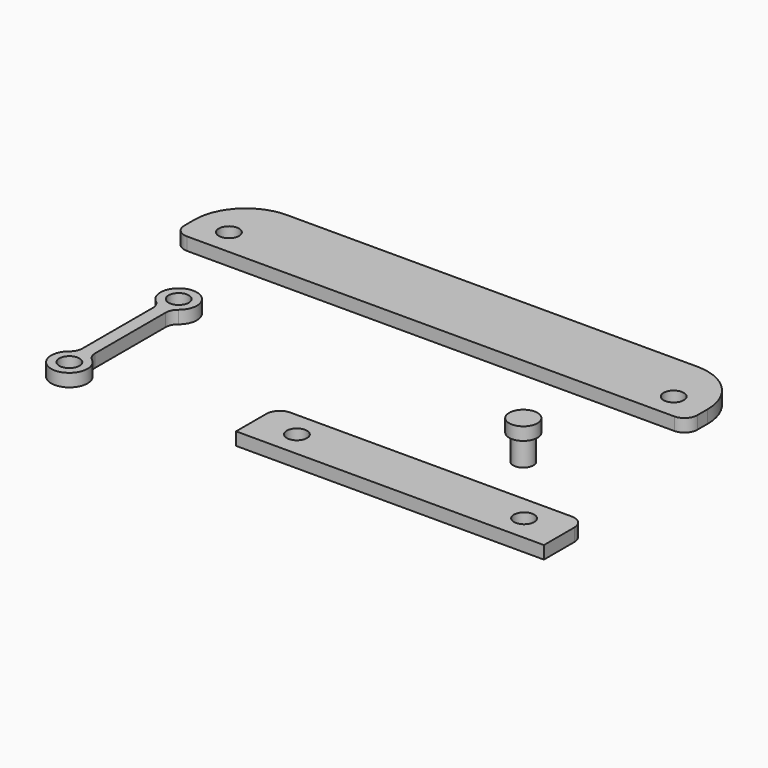
from build123d import *

# Parameters (mm, degrees)
F0_R     = 2.5
F1_DEPTH = 3.175
F2_R     = 2.5
F3_DEPTH = 3.175
F4_R     = 2.5
F5_DEPTH = 6.35
F4_R_2   = 3.5
F6_DEPTH = 3.175
F8_DEPTH = 3.175


# Not quite as in the source:
# - a length typed as a fraction of an inch, garbled in the dataset ("3 / 203.2 mm" for 3/8 in), is restored


with BuildPart() as f1:
    # F0 (on Top) → F1 (new body)
    with BuildSketch(Plane.XY):
        with BuildLine():
            ThreePointArc((-33.712554723, 10.891355979), (-33.3953284467, 12.2747410823), (-32.5070401756, 13.3816876943))
            ThreePointArc((-32.5070401756, 13.3816876943), (-35.2984368801, 21.4112917002), (-38.0898335846, 13.3816876943))
            ThreePointArc((-38.0898335846, 13.3816876943), (-37.2015453135, 12.2747410823), (-36.8843190372, 10.891355979))
            Line((-36.8843190372, 10.891355979), (-36.8843190372, 0))
            Line((-36.8843190372, 0), (-33.712554723, 0))
            Line((-33.712554723, 0), (-33.712554723, 10.891355979))
        make_face()
        with Locations((-35.2984368801, 16.9112917002)):
            Circle(F0_R, mode=Mode.SUBTRACT)
        with BuildLine():
            Line((-33.712554723, -10.891355979), (-33.712554723, 0))
            Line((-33.712554723, 0), (-36.8843190372, 0))
            Line((-36.8843190372, 0), (-36.8843190372, -10.891355979))
            ThreePointArc((-36.8843190372, -10.891355979), (-37.2015453135, -12.2747410823), (-38.0898335846, -13.3816876943))
            ThreePointArc((-38.0898335846, -13.3816876943), (-35.2984368801, -21.4112917002), (-32.5070401756, -13.3816876943))
            ThreePointArc((-32.5070401756, -13.3816876943), (-33.3953284467, -12.2747410823), (-33.712554723, -10.891355979))
        make_face()
        with Locations((-35.2984368801, -16.9112917002)):
            Circle(F0_R, mode=Mode.SUBTRACT)
    extrude(amount=F1_DEPTH)


with BuildPart() as f3:
    # F2 (on Top) → F3 (new body)
    with BuildSketch(Plane.XY):
        with BuildLine():
            ThreePointArc((-53.6429062486, 41.5569074162), (-52.7129702788, 39.3118433859), (-50.4679062486, 38.3819074162))
            Line((-50.4679062486, 38.3819074162), (9.8570937514, 38.3819074162))
            Line((9.8570937514, 38.3819074162), (70.1820937514, 38.3819074162))
            ThreePointArc((70.1820937514, 38.3819074162), (72.4271577817, 39.3118433859), (73.3570937514, 41.5569074162))
            Line((73.3570937514, 41.5569074162), (73.3570937514, 44.7319074162))
            ThreePointArc((73.3570937514, 44.7319074162), (69.6373498725, 53.7121635373), (60.6570937514, 57.4319074162))
            Line((60.6570937514, 57.4319074162), (9.8570937514, 57.4319074162))
            Line((9.8570937514, 57.4319074162), (-40.9429062486, 57.4319074162))
            ThreePointArc((-40.9429062486, 57.4319074162), (-49.9231623696, 53.7121635373), (-53.6429062486, 44.7319074162))
            Line((-53.6429062486, 44.7319074162), (-53.6429062486, 41.5569074162))
        make_face()
        with Locations((-45.1785493704, 44.8088147985)):
            Circle(F2_R, mode=Mode.SUBTRACT)
        with Locations((64.8927368733, 44.8088147985)):
            Circle(F2_R, mode=Mode.SUBTRACT)
    extrude(amount=F3_DEPTH)


with BuildPart() as f5:
    # F4 (on Top) → F5 (new body)
    with BuildSketch(Plane.XY):
        with Locations((47.8275045753, 19.6292065084)):
            Circle(F4_R)
    extrude(amount=-F5_DEPTH)

    # F4 (on Top) → F6 (join)
    with BuildSketch(Plane.XY):
        with Locations((47.8275045753, 19.6292065084)):
            Circle(F4_R_2)
        with Locations((47.8275045753, 19.6292065084)):
            Circle(F4_R, mode=Mode.SUBTRACT)
        with Locations((47.8275045753, 19.6292065084)):
            Circle(F4_R)
    extrude(amount=F6_DEPTH)


with BuildPart() as f8:
    # F7 (on Top) → F8 (new body)
    with BuildSketch(Plane.XY):
        with BuildLine():
            Line((46.0545447382, -6.708232842), (11.2443861502, -6.708232842))
            ThreePointArc((11.2443861502, -6.708232842), (8.9181169788, -7.6718050825), (7.9545447382, -9.9980742539))
            Line((7.9545447382, -9.9980742539), (7.9545447382, -19.408232842))
            Line((7.9545447382, -19.408232842), (17.9369021207, -19.408232842))
            Line((17.9369021207, -19.408232842), (46.0545447382, -19.408232842))
            Line((46.0545447382, -19.408232842), (74.1721873558, -19.408232842))
            Line((74.1721873558, -19.408232842), (84.1545447382, -19.408232842))
            Line((84.1545447382, -19.408232842), (84.1545447382, -9.9980742539))
            ThreePointArc((84.1545447382, -9.9980742539), (83.1909724977, -7.6718050825), (80.8647033263, -6.708232842))
            Line((80.8647033263, -6.708232842), (46.0545447382, -6.708232842))
        make_face()
        with BuildLine():
            ThreePointArc((20.4369021207, -13.058232842), (19.7046690737, -14.825999795), (17.9369021207, -15.558232842))
            ThreePointArc((17.9369021207, -15.558232842), (16.1691351677, -11.290465889), (20.4369021207, -13.058232842))
        make_face(mode=Mode.SUBTRACT)
        with BuildLine():
            ThreePointArc((76.6721873558, -13.058232842), (75.9399543087, -14.825999795), (74.1721873558, -15.558232842))
            ThreePointArc((74.1721873558, -15.558232842), (72.4044204028, -11.290465889), (76.6721873558, -13.058232842))
        make_face(mode=Mode.SUBTRACT)
    extrude(amount=F8_DEPTH)


solid = Compound([f1.part, f3.part, f5.part, f8.part])
